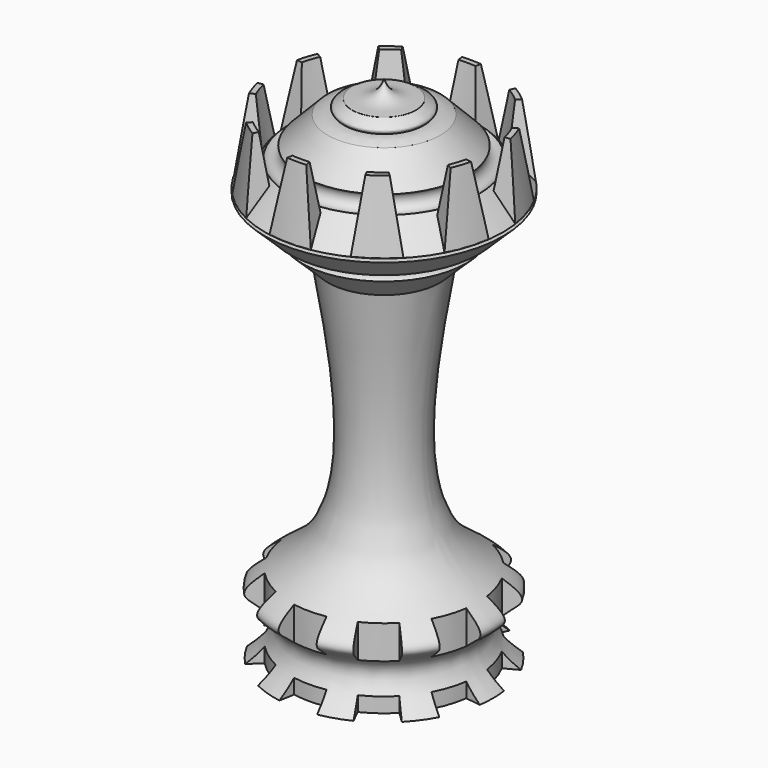
from build123d import *

# Parameters (mm, degrees)
F5_DEPTH                  = 8
DRAFT_F5_DRAFTED_ANGLE    = 8
DRAFT_F5_2_DRAFTED_ANGLE  = 8
DRAFT_F5_3_DRAFTED_ANGLE  = 8
DRAFT_F5_4_DRAFTED_ANGLE  = 8
DRAFT_F5_5_DRAFTED_ANGLE  = 8
DRAFT_F5_6_DRAFTED_ANGLE  = 8
DRAFT_F5_7_DRAFTED_ANGLE  = 8
DRAFT_F5_8_DRAFTED_ANGLE  = 8
DRAFT_F5_9_DRAFTED_ANGLE  = 8
DRAFT_F5_10_DRAFTED_ANGLE = 8
F6_DEPTH                  = 10


# Not quite as in the source:
# - an extrude with a draft is written as a straight extrude whose walls are then drafted


with BuildPart() as f1:
    # F0 (on Front) → F1 (revolve)
    with BuildSketch(Plane.XZ):
        with BuildLine():
            Line((0, 60), (0, 0))
            Line((0, 0), (12.7955756747, 0))
            add(Edge.make_bspline(
                [(12.7955756747, 0), (7.225355003, 4.5141381884), (17.1439867692, 6.9535461926), (2.4609813912, 12.2450062723), (4.3828166152, 28.3329467463), (6.6034411258, 40.9907293966)],
                knots=[0, 0, 0, 0, 0.2456110483, 0.5014802111, 1, 1, 1, 1], degree=3))
            Line((6.6034411258, 40.9907293966), (9.6957204404, 44.0042307699))
            ThreePointArc((9.6957204404, 44.0042307699), (9.7139653737, 45.4183266374), (11.1280612412, 45.4000817041))
            Line((11.1280612412, 45.4000817041), (14.0054894357, 48.2042054373))
            Line((14.0054894357, 48.2042054373), (12.7288400681, 48.4135830774))
            Line((12.7288400681, 48.4135830774), (14.0109629156, 48.6284341975))
            Line((14.0109629156, 48.6284341975), (11.1098163079, 51.605421606))
            ThreePointArc((11.1098163079, 51.605421606), (9.6957204404, 51.6236665393), (9.7139653737, 53.0377624068))
            Line((9.7139653737, 53.0377624068), (6.6034411258, 56.2296009354))
            add(Edge.make_bspline(
                [(6.6034411258, 56.2296009354), (3.8324046692, 56.0041256272), (-1.1945774341, 55.337696937), (3.737609173, 57.6859205172), (3.7362605799, 57.9154714942)],
                knots=[0, 0, 0, 0, 0.3776826062, 0.6594548857, 0.6594548857, 0.6594548857, 0.6594548857], degree=3))
            add(Edge.make_bspline(
                [(3.7362605799, 57.9154714942), (3.7346306936, 58.1929028435), (0.6527698715, 57.34006688), (0, 60)],
                knots=[0.6594548857, 0.6594548857, 0.6594548857, 0.6594548857, 1, 1, 1, 1], degree=3))
        make_face()
        with BuildLine():
            add(Edge.make_bspline(
                [(3.7362605799, 57.9154714942), (4.2966801861, 57.6297486487), (5.0678420216, 57.236581544), (4.8117730145, 56.7830649444), (4.6937745736, 56.6563072724)],
                knots=[0, 0, 0, 0, 0.4986670914, 0.6861876802, 0.6861876802, 0.6861876802, 0.6861876802], degree=3))
            add(Edge.make_bspline(
                [(6.6034411258, 56.2296009354), (3.8324046692, 56.0041256272), (-1.1945774341, 55.337696937), (3.737609173, 57.6859205172), (3.7362605799, 57.9154714942)],
                knots=[0, 0, 0, 0, 0.3776826062, 0.6594548857, 0.6594548857, 0.6594548857, 0.6594548857], degree=3))
            add(Edge.make_bspline(
                [(4.6937745736, 56.6563072724), (4.9792195966, 56.6651731858), (5.5874586713, 56.6832227704), (6.2513988471, 56.3868645305), (6.6034411258, 56.2296009354)],
                knots=[0, 0, 0, 0, 0.46976271, 1, 1, 1, 1], degree=3))
        make_face()
    revolve(axis=Axis((0, 0, 30), (0, 0, 1)))


with BuildPart() as f5_drafted:
    # F4 (on offset) → F5 (new body)
    with BuildSketch(Plane.XY.offset(48.62)):
        with BuildLine():
            Line((1.9296717203, 10.9437121454), (2.4310744873, 13.7873085422))
            ThreePointArc((2.4310744873, 13.7873085422), (0, 14), (-2.4310744873, 13.7873085422))
            Line((-2.4310744873, 13.7873085422), (-1.9296717203, 10.9437121454))
            ThreePointArc((-1.9296717203, 10.9437121454), (0, 11.1125365452), (1.9296717203, 10.9437121454))
        make_face()
    extrude(amount=F5_DEPTH)

    # draft_F5_drafted
    draft_f5_drafted_walls = [f5_drafted.faces().sort_by_distance(p)[0] for p in [
        (0, 14, 53.9533333333),
        (-2.1803731038, 12.3655103438, 53.9533333333),
        (0, 11.1125365452, 53.9533333333),
        (2.1803731038, 12.3655103438, 53.9533333333),
    ]]
    draft(draft_f5_drafted_walls, neutral_plane=Plane.XY.offset(48.62), angle=DRAFT_F5_DRAFTED_ANGLE)


with BuildPart() as f1_1:
    add(f1.part)

    # join_F5_drafted: union F5_drafted
    add(f5_drafted.part)


with BuildPart() as f5_2_drafted:
    # F4 (on offset) → F5, piece 2 (new body)
    with BuildSketch(Plane.XY.offset(48.62)):
        with BuildLine():
            Line((-4.8714153891, 9.9878816861), (-6.137196055, 12.5831166482))
            ThreePointArc((-6.137196055, 12.5831166482), (-8.2289935321, 11.3262379212), (-10.0707572047, 9.7252171864))
            Line((-10.0707572047, 9.7252171864), (-7.9936898197, 7.7194165282))
            ThreePointArc((-7.9936898197, 7.7194165282), (-6.5317850968, 8.9902309157), (-4.8714153891, 9.9878816861))
        make_face()
    extrude(amount=F5_DEPTH)

    # draft_F5_2_drafted
    draft_f5_2_drafted_walls = [f5_2_drafted.faces().sort_by_distance(p)[0] for p in [
        (-8.2289935321, 11.3262379212, 53.9533333333),
        (-9.0322235122, 8.7223168573, 53.9533333333),
        (-6.5317850968, 8.9902309157, 53.9533333333),
        (-5.5043057221, 11.2854991672, 53.9533333333),
    ]]
    draft(draft_f5_2_drafted_walls, neutral_plane=Plane.XY.offset(48.62), angle=DRAFT_F5_2_DRAFTED_ANGLE)


with BuildPart() as f1_2:
    add(f1_1.part)

    # join_F5_2_drafted: union F5_2_drafted
    add(f5_2_drafted.part)


with BuildPart() as f5_3_drafted:
    # F4 (on offset) → F5, piece 3 (new body)
    with BuildSketch(Plane.XY.offset(48.62)):
        with BuildLine():
            Line((-9.8117873932, 5.2170198984), (-12.3612663, 6.572601879))
            ThreePointArc((-12.3612663, 6.572601879), (-13.3147912281, 4.3262379212), (-13.8637529624, 1.9484234134))
            Line((-13.8637529624, 1.9484234134), (-11.0043901035, 1.5465661705))
            ThreePointArc((-11.0043901035, 1.5465661705), (-10.5686502939, 3.4339626431), (-9.8117873932, 5.2170198984))
        make_face()
    extrude(amount=F5_DEPTH)

    # draft_F5_3_drafted
    draft_f5_3_drafted_walls = [f5_3_drafted.faces().sort_by_distance(p)[0] for p in [
        (-10.5686502939, 3.4339626431, 53.9533333333),
        (-11.0865268466, 5.8948108887, 53.9533333333),
        (-13.3147912281, 4.3262379212, 53.9533333333),
        (-12.4340715329, 1.747494792, 53.9533333333),
    ]]
    draft(draft_f5_3_drafted_walls, neutral_plane=Plane.XY.offset(48.62), angle=DRAFT_F5_3_DRAFTED_ANGLE)


with BuildPart() as f1_3:
    add(f1_2.part)

    # join_F5_3_drafted: union F5_3_drafted
    add(f5_3_drafted.part)


with BuildPart() as f5_4_drafted:
    # F4 (on offset) → F5, piece 4 (new body)
    with BuildSketch(Plane.XY.offset(48.62)):
        with BuildLine():
            Line((-11.0043901035, -1.5465661705), (-13.8637529624, -1.9484234134))
            ThreePointArc((-13.8637529624, -1.9484234134), (-13.3147912281, -4.3262379212), (-12.3612663, -6.572601879))
            Line((-12.3612663, -6.572601879), (-9.8117873932, -5.2170198984))
            ThreePointArc((-9.8117873932, -5.2170198984), (-10.5686502939, -3.4339626431), (-11.0043901035, -1.5465661705))
        make_face()
    extrude(amount=F5_DEPTH)

    # draft_F5_4_drafted
    draft_f5_4_drafted_walls = [f5_4_drafted.faces().sort_by_distance(p)[0] for p in [
        (-11.0865268466, -5.8948108887, 53.9533333333),
        (-10.5686502939, -3.4339626431, 53.9533333333),
        (-12.4340715329, -1.747494792, 53.9533333333),
        (-13.3147912281, -4.3262379212, 53.9533333333),
    ]]
    draft(draft_f5_4_drafted_walls, neutral_plane=Plane.XY.offset(48.62), angle=DRAFT_F5_4_DRAFTED_ANGLE)


with BuildPart() as f1_4:
    add(f1_3.part)

    # join_F5_4_drafted: union F5_4_drafted
    add(f5_4_drafted.part)


with BuildPart() as f5_5_drafted:
    # F4 (on offset) → F5, piece 5 (new body)
    with BuildSketch(Plane.XY.offset(48.62)):
        with BuildLine():
            Line((-7.9936898197, -7.7194165282), (-10.0707572047, -9.7252171864))
            ThreePointArc((-10.0707572047, -9.7252171864), (-8.2289935321, -11.3262379212), (-6.137196055, -12.5831166482))
            Line((-6.137196055, -12.5831166482), (-4.8714153891, -9.9878816861))
            ThreePointArc((-4.8714153891, -9.9878816861), (-6.5317850968, -8.9902309157), (-7.9936898197, -7.7194165282))
        make_face()
    extrude(amount=F5_DEPTH)

    # draft_F5_5_drafted
    draft_f5_5_drafted_walls = [f5_5_drafted.faces().sort_by_distance(p)[0] for p in [
        (-8.2289935321, -11.3262379212, 53.9533333333),
        (-5.5043057221, -11.2854991672, 53.9533333333),
        (-6.5317850968, -8.9902309157, 53.9533333333),
        (-9.0322235122, -8.7223168573, 53.9533333333),
    ]]
    draft(draft_f5_5_drafted_walls, neutral_plane=Plane.XY.offset(48.62), angle=DRAFT_F5_5_DRAFTED_ANGLE)


with BuildPart() as f1_5:
    add(f1_4.part)

    # join_F5_5_drafted: union F5_5_drafted
    add(f5_5_drafted.part)


with BuildPart() as f5_6_drafted:
    # F4 (on offset) → F5, piece 6 (new body)
    with BuildSketch(Plane.XY.offset(48.62)):
        with BuildLine():
            Line((-1.9296717203, -10.9437121454), (-2.4310744873, -13.7873085422))
            ThreePointArc((-2.4310744873, -13.7873085422), (0, -14), (2.4310744873, -13.7873085422))
            Line((2.4310744873, -13.7873085422), (1.9296717203, -10.9437121454))
            ThreePointArc((1.9296717203, -10.9437121454), (0, -11.1125365452), (-1.9296717203, -10.9437121454))
        make_face()
    extrude(amount=F5_DEPTH)

    # draft_F5_6_drafted
    draft_f5_6_drafted_walls = [f5_6_drafted.faces().sort_by_distance(p)[0] for p in [
        (2.1803731038, -12.3655103438, 53.9533333333),
        (0, -11.1125365452, 53.9533333333),
        (-2.1803731038, -12.3655103438, 53.9533333333),
        (0, -14, 53.9533333333),
    ]]
    draft(draft_f5_6_drafted_walls, neutral_plane=Plane.XY.offset(48.62), angle=DRAFT_F5_6_DRAFTED_ANGLE)


with BuildPart() as f1_6:
    add(f1_5.part)

    # join_F5_6_drafted: union F5_6_drafted
    add(f5_6_drafted.part)


with BuildPart() as f5_7_drafted:
    # F4 (on offset) → F5, piece 7 (new body)
    with BuildSketch(Plane.XY.offset(48.62)):
        with BuildLine():
            Line((4.8714153891, -9.9878816861), (6.137196055, -12.5831166482))
            ThreePointArc((6.137196055, -12.5831166482), (8.2289935321, -11.3262379212), (10.0707572047, -9.7252171864))
            Line((10.0707572047, -9.7252171864), (7.9936898197, -7.7194165282))
            ThreePointArc((7.9936898197, -7.7194165282), (6.5317850968, -8.9902309157), (4.8714153891, -9.9878816861))
        make_face()
    extrude(amount=F5_DEPTH)

    # draft_F5_7_drafted
    draft_f5_7_drafted_walls = [f5_7_drafted.faces().sort_by_distance(p)[0] for p in [
        (6.5317850968, -8.9902309157, 53.9533333333),
        (5.5043057221, -11.2854991672, 53.9533333333),
        (8.2289935321, -11.3262379212, 53.9533333333),
        (9.0322235122, -8.7223168573, 53.9533333333),
    ]]
    draft(draft_f5_7_drafted_walls, neutral_plane=Plane.XY.offset(48.62), angle=DRAFT_F5_7_DRAFTED_ANGLE)


with BuildPart() as f1_7:
    add(f1_6.part)

    # join_F5_7_drafted: union F5_7_drafted
    add(f5_7_drafted.part)


with BuildPart() as f5_8_drafted:
    # F4 (on offset) → F5, piece 8 (new body)
    with BuildSketch(Plane.XY.offset(48.62)):
        with BuildLine():
            Line((9.8117873932, -5.2170198984), (12.3612663, -6.572601879))
            ThreePointArc((12.3612663, -6.572601879), (13.3147912281, -4.3262379212), (13.8637529624, -1.9484234134))
            Line((13.8637529624, -1.9484234134), (11.0043901035, -1.5465661705))
            ThreePointArc((11.0043901035, -1.5465661705), (10.5686502939, -3.4339626431), (9.8117873932, -5.2170198984))
        make_face()
    extrude(amount=F5_DEPTH)

    # draft_F5_8_drafted
    draft_f5_8_drafted_walls = [f5_8_drafted.faces().sort_by_distance(p)[0] for p in [
        (13.3147912281, -4.3262379212, 53.9533333333),
        (12.4340715329, -1.747494792, 53.9533333333),
        (10.5686502939, -3.4339626431, 53.9533333333),
        (11.0865268466, -5.8948108887, 53.9533333333),
    ]]
    draft(draft_f5_8_drafted_walls, neutral_plane=Plane.XY.offset(48.62), angle=DRAFT_F5_8_DRAFTED_ANGLE)


with BuildPart() as f1_8:
    add(f1_7.part)

    # join_F5_8_drafted: union F5_8_drafted
    add(f5_8_drafted.part)


with BuildPart() as f5_9_drafted:
    # F4 (on offset) → F5, piece 9 (new body)
    with BuildSketch(Plane.XY.offset(48.62)):
        with BuildLine():
            Line((11.0043901035, 1.5465661705), (13.8637529624, 1.9484234134))
            ThreePointArc((13.8637529624, 1.9484234134), (13.3147912281, 4.3262379212), (12.3612663, 6.572601879))
            Line((12.3612663, 6.572601879), (9.8117873932, 5.2170198984))
            ThreePointArc((9.8117873932, 5.2170198984), (10.5686502939, 3.4339626431), (11.0043901035, 1.5465661705))
        make_face()
    extrude(amount=F5_DEPTH)

    # draft_F5_9_drafted
    draft_f5_9_drafted_walls = [f5_9_drafted.faces().sort_by_distance(p)[0] for p in [
        (10.5686502939, 3.4339626431, 53.9533333333),
        (12.4340715329, 1.747494792, 53.9533333333),
        (13.3147912281, 4.3262379212, 53.9533333333),
        (11.0865268466, 5.8948108887, 53.9533333333),
    ]]
    draft(draft_f5_9_drafted_walls, neutral_plane=Plane.XY.offset(48.62), angle=DRAFT_F5_9_DRAFTED_ANGLE)


with BuildPart() as f1_9:
    add(f1_8.part)

    # join_F5_9_drafted: union F5_9_drafted
    add(f5_9_drafted.part)


with BuildPart() as f5_10_drafted:
    # F4 (on offset) → F5, piece 10 (new body)
    with BuildSketch(Plane.XY.offset(48.62)):
        with BuildLine():
            Line((7.9936898197, 7.7194165282), (10.0707572047, 9.7252171864))
            ThreePointArc((10.0707572047, 9.7252171864), (8.2289935321, 11.3262379212), (6.137196055, 12.5831166482))
            Line((6.137196055, 12.5831166482), (4.8714153891, 9.9878816861))
            ThreePointArc((4.8714153891, 9.9878816861), (6.5317850968, 8.9902309157), (7.9936898197, 7.7194165282))
        make_face()
    extrude(amount=F5_DEPTH)

    # draft_F5_10_drafted
    draft_f5_10_drafted_walls = [f5_10_drafted.faces().sort_by_distance(p)[0] for p in [
        (5.5043057221, 11.2854991672, 53.9533333333),
        (6.5317850968, 8.9902309157, 53.9533333333),
        (9.0322235122, 8.7223168573, 53.9533333333),
        (8.2289935321, 11.3262379212, 53.9533333333),
    ]]
    draft(draft_f5_10_drafted_walls, neutral_plane=Plane.XY.offset(48.62), angle=DRAFT_F5_10_DRAFTED_ANGLE)


with BuildPart() as f1_10:
    add(f1_9.part)

    # join_F5_10_drafted: union F5_10_drafted
    add(f5_10_drafted.part)

    # F2 (on Top) → F6 (cut)
    with BuildSketch(Plane.XY):
        with BuildLine():
            ThreePointArc((-2.4310744873, -13.7873085422), (0, -14), (2.4310744873, -13.7873085422))
            Line((2.4310744873, -13.7873085422), (1.9101299543, -10.8328852831))
            ThreePointArc((1.9101299543, -10.8328852831), (0, -11), (-1.9101299543, -10.8328852831))
            Line((-1.9101299543, -10.8328852831), (-2.4310744873, -13.7873085422))
        make_face()
        with BuildLine():
            Line((4.8220826147, -9.8867345093), (6.137196055, -12.5831166482))
            ThreePointArc((6.137196055, -12.5831166482), (8.2289935321, -11.3262379212), (10.0707572047, -9.7252171864))
            Line((10.0707572047, -9.7252171864), (7.9127378037, -7.641242075))
            ThreePointArc((7.9127378037, -7.641242075), (6.4656377752, -8.8991869381), (4.8220826147, -9.8867345093))
        make_face()
        with BuildLine():
            Line((9.7124235214, -5.1641871906), (12.3612663, -6.572601879))
            ThreePointArc((12.3612663, -6.572601879), (13.3147912281, -4.3262379212), (13.8637529624, -1.9484234134))
            Line((13.8637529624, -1.9484234134), (10.8929487562, -1.5309041106))
            ThreePointArc((10.8929487562, -1.5309041106), (10.4616216792, -3.3991869381), (9.7124235214, -5.1641871906))
        make_face()
        with BuildLine():
            Line((10.8929487562, 1.5309041106), (13.8637529624, 1.9484234134))
            ThreePointArc((13.8637529624, 1.9484234134), (13.3147912281, 4.3262379212), (12.3612663, 6.572601879))
            Line((12.3612663, 6.572601879), (9.7124235214, 5.1641871906))
            ThreePointArc((9.7124235214, 5.1641871906), (10.4616216792, 3.3991869381), (10.8929487562, 1.5309041106))
        make_face()
        with BuildLine():
            Line((7.9127378037, 7.641242075), (10.0707572047, 9.7252171864))
            ThreePointArc((10.0707572047, 9.7252171864), (8.2289935321, 11.3262379212), (6.137196055, 12.5831166482))
            Line((6.137196055, 12.5831166482), (4.8220826147, 9.8867345093))
            ThreePointArc((4.8220826147, 9.8867345093), (6.4656377752, 8.8991869381), (7.9127378037, 7.641242075))
        make_face()
        with BuildLine():
            Line((1.9101299543, 10.8328852831), (2.4310744873, 13.7873085422))
            ThreePointArc((2.4310744873, 13.7873085422), (0, 14), (-2.4310744873, 13.7873085422))
            Line((-2.4310744873, 13.7873085422), (-1.9101299543, 10.8328852831))
            ThreePointArc((-1.9101299543, 10.8328852831), (0, 11), (1.9101299543, 10.8328852831))
        make_face()
        with BuildLine():
            Line((-4.8220826147, 9.8867345093), (-6.137196055, 12.5831166482))
            ThreePointArc((-6.137196055, 12.5831166482), (-8.2289935321, 11.3262379212), (-10.0707572047, 9.7252171864))
            Line((-10.0707572047, 9.7252171864), (-7.9127378037, 7.641242075))
            ThreePointArc((-7.9127378037, 7.641242075), (-6.4656377752, 8.8991869381), (-4.8220826147, 9.8867345093))
        make_face()
        with BuildLine():
            Line((-9.7124235214, 5.1641871906), (-12.3612663, 6.572601879))
            ThreePointArc((-12.3612663, 6.572601879), (-13.3147912281, 4.3262379212), (-13.8637529624, 1.9484234134))
            Line((-13.8637529624, 1.9484234134), (-10.8929487562, 1.5309041106))
            ThreePointArc((-10.8929487562, 1.5309041106), (-10.4616216792, 3.3991869381), (-9.7124235214, 5.1641871906))
        make_face()
        with BuildLine():
            Line((-10.8929487562, -1.5309041106), (-13.8637529624, -1.9484234134))
            ThreePointArc((-13.8637529624, -1.9484234134), (-13.3147912281, -4.3262379212), (-12.3612663, -6.572601879))
            Line((-12.3612663, -6.572601879), (-9.7124235214, -5.1641871906))
            ThreePointArc((-9.7124235214, -5.1641871906), (-10.4616216792, -3.3991869381), (-10.8929487562, -1.5309041106))
        make_face()
        with BuildLine():
            Line((-7.9127378037, -7.641242075), (-10.0707572047, -9.7252171864))
            ThreePointArc((-10.0707572047, -9.7252171864), (-8.2289935321, -11.3262379212), (-6.137196055, -12.5831166482))
            Line((-6.137196055, -12.5831166482), (-4.8220826147, -9.8867345093))
            ThreePointArc((-4.8220826147, -9.8867345093), (-6.4656377752, -8.8991869381), (-7.9127378037, -7.641242075))
        make_face()
    extrude(amount=F6_DEPTH, mode=Mode.SUBTRACT)


solid = f1_10.part
